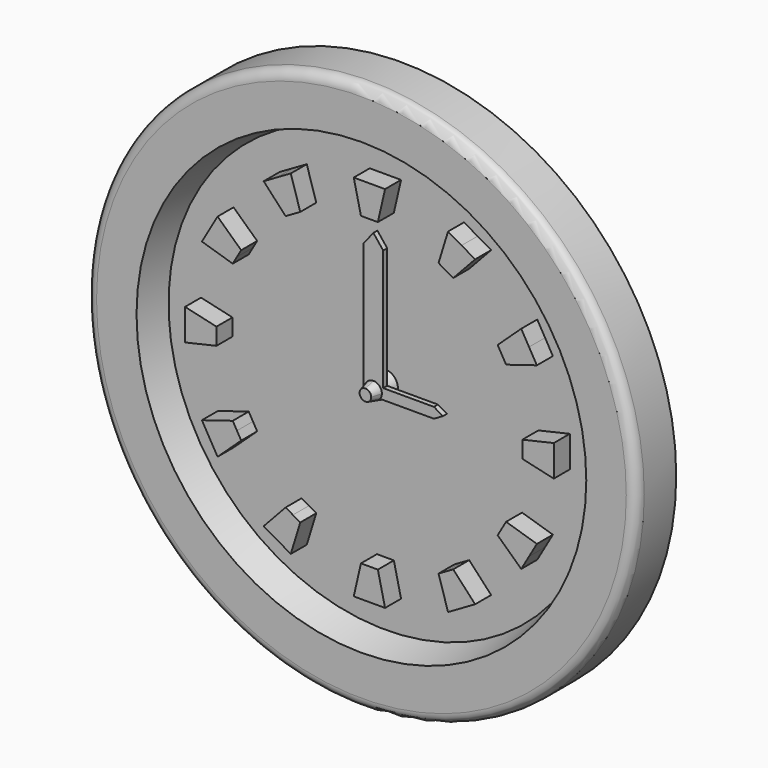
from build123d import *

# Parameters (mm, degrees)
F0_R      = 55
F1_DEPTH  = 10
F2_R      = 45
F3_DEPTH  = 6
F3_TAPER  = 15
F5_DEPTH  = 4
F11_DEPTH = 5
F11_TAPER = 15
F14_DEPTH = 1
F16_DEPTH = 1
F17_R     = 2


# Not quite as in the source:
# - the program builds the solid bodies; features that only make, move or delete a surface that nothing else refers to are left out


with BuildPart() as f1:
    # F0 (on Front) → F1 (new body)
    with BuildSketch(Plane.XZ):
        Circle(F0_R)
    extrude(amount=F1_DEPTH)

    # F2 (on face) → F3 (cut)
    with BuildSketch(Plane.XZ.offset(10)):
        Circle(F2_R)
    extrude(amount=-F3_DEPTH, taper=F3_TAPER, mode=Mode.SUBTRACT)

    # F4 (on face) → F5 (join)
    with BuildSketch(Plane.XZ.offset(4)):
        Polygon((0, 36.8904769421), (-3.1339118723, 36.8904769421), (-1.6905769007, 30.6056980044), (0, 30.6056980044), (1.6905769007, 30.6056980044), (3.1339118723, 36.8904769421), align=None)
        Polygon((18.445238471, 31.9480901896), (15.7311911764, 33.5150461257), (13.8387664591, 27.3506004227), (15.3028490022, 26.5053119723), (16.7669315453, 25.660023522), (21.1592857656, 30.3811342534), align=None)
        Polygon((31.9480901896, 18.445238471), (30.3811342534, 21.1592857656), (25.660023522, 16.7669315453), (26.5053119723, 15.3028490022), (27.3506004227, 13.8387664591), (33.5150461257, 15.7311911764), align=None)
        Polygon((36.8904769421, 0), (36.8904769421, 3.1339118723), (30.6056980044, 1.6905769007), (30.6056980044, 0), (30.6056980044, -1.6905769007), (36.8904769421, -3.1339118723), align=None)
        Polygon((31.9480901896, -18.445238471), (33.5150461257, -15.7311911764), (27.3506004227, -13.8387664591), (26.5053119723, -15.3028490022), (25.660023522, -16.7669315453), (30.3811342534, -21.1592857656), align=None)
        Polygon((18.445238471, -31.9480901896), (21.1592857656, -30.3811342534), (16.7669315453, -25.660023522), (15.3028490022, -26.5053119723), (13.8387664591, -27.3506004227), (15.7311911764, -33.5150461257), align=None)
        Polygon((0, -36.8904769421), (3.1339118723, -36.8904769421), (1.6905769007, -30.6056980044), (0, -30.6056980044), (-1.6905769007, -30.6056980044), (-3.1339118723, -36.8904769421), align=None)
        Polygon((-18.445238471, -31.9480901896), (-15.7311911764, -33.5150461257), (-13.8387664591, -27.3506004227), (-15.3028490022, -26.5053119723), (-16.7669315453, -25.660023522), (-21.1592857656, -30.3811342534), align=None)
        Polygon((-31.9480901896, -18.445238471), (-30.3811342534, -21.1592857656), (-25.660023522, -16.7669315453), (-26.5053119723, -15.3028490022), (-27.3506004227, -13.8387664591), (-33.5150461257, -15.7311911764), align=None)
        Polygon((-36.8904769421, 0), (-36.8904769421, -3.1339118723), (-30.6056980044, -1.6905769007), (-30.6056980044, 0), (-30.6056980044, 1.6905769007), (-36.8904769421, 3.1339118723), align=None)
        Polygon((-31.9480901896, 18.445238471), (-33.5150461257, 15.7311911764), (-27.3506004227, 13.8387664591), (-26.5053119723, 15.3028490022), (-25.660023522, 16.7669315453), (-30.3811342534, 21.1592857656), align=None)
        Polygon((-18.445238471, 31.9480901896), (-21.1592857656, 30.3811342534), (-16.7669315453, 25.660023522), (-15.3028490022, 26.5053119723), (-13.8387664591, 27.3506004227), (-15.7311911764, 33.5150461257), align=None)
    extrude(amount=F5_DEPTH)

    # F17
    f17_edges = [f1.edges().sort_by_distance(p)[0] for p in [
        (-55, -10, 0),
    ]]
    fillet(f17_edges, radius=F17_R)


with BuildPart() as f11:
    # F10 (on offset) → F11 (new body)
    with BuildSketch(Plane.XZ.offset(4)):
        with BuildLine():
            ThreePointArc((0, -2.5), (1.767766953, -1.767766953), (2.5, 0))
            ThreePointArc((2.5, 0), (1.767766953, 1.767766953), (0, 2.5))
            Line((0, 2.5), (0, -2.5))
        make_face()
        with BuildLine():
            Line((0, -2.5), (0, 2.5))
            ThreePointArc((0, 2.5), (-2.5, 0), (0, -2.5))
        make_face()
    extrude(amount=F11_DEPTH, taper=F11_TAPER)

    # F13 (on offset) → F14 (join)
    with BuildSketch(Plane.XZ.offset(6)):
        Polygon((0, 27.7616046369), (-1.9594193436, 25.2858418971), (0, 25.2858418971), (1.9594193436, 25.2858418971), align=None)
        Polygon((0, 25.2858418971), (-1.9594193436, 25.2858418971), (-1.9594193436, 0), (1.9594193436, 0), (1.9594193436, 25.2858418971), align=None)
    extrude(amount=F14_DEPTH)

    # F15 (on offset) → F16 (join)
    with BuildSketch(Plane.XZ.offset(6)):
        Polygon((12.1070826426, 0), (12.1070826426, 1.0465652449), (0, 1.0465652449), (0, -1.0465652449), (12.1070826426, -1.0465652449), align=None)
        Polygon((13.9101780951, 0), (12.1070826426, 1.0465652449), (12.1070826426, 0), (12.1070826426, -1.0465652449), align=None)
    extrude(amount=F16_DEPTH)


solid = Compound([f1.part, f11.part])
